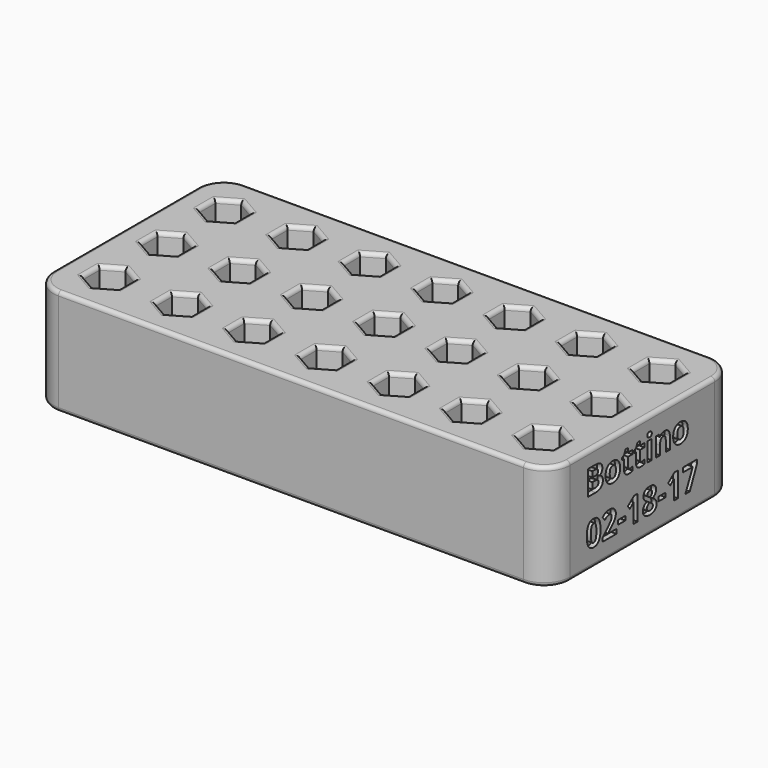
from build123d import *

# Parameters (mm, degrees)
F2_DEPTH     = 20.5
F3_DEPTH     = 12
F4_DEPTH     = 17
F5_R         = 0.5
F6_R         = 0.75
F7_TEXT_SIZE = 6.6788283418
F8_DEPTH     = 1


# Not quite as in the source:
# - Text() gives the source's letters only with a copy of the font that has no kerning and outlines rounded to 1/6400 em; it was checked with that copy


with BuildPart() as f2:
    # F1 (on Top) → F2 (new body)
    with BuildSketch(Plane.XY):
        with BuildLine():
            Line((45, 22.5), (-45, 22.5))
            ThreePointArc((-45, 22.5), (-48.5355339059, 21.0355339059), (-50, 17.5))
            Line((-50, 17.5), (-50, -17.5))
            ThreePointArc((-50, -17.5), (-48.5355339059, -21.0355339059), (-45, -22.5))
            Line((-45, -22.5), (45, -22.5))
            ThreePointArc((45, -22.5), (48.5355339059, -21.0355339059), (50, -17.5))
            Line((50, -17.5), (50, 17.5))
            ThreePointArc((50, 17.5), (48.5355339059, 21.0355339059), (45, 22.5))
        make_face()
    extrude(amount=-F2_DEPTH)

    # F0 (on Top) → F3 (cut)
    with BuildSketch(Plane.XY):
        Polygon((-42, -10.0451506561), (-45.425, -12.022575328), (-45.425, -15.977424672), (-42, -17.9548493439), (-38.575, -15.977424672), (-38.575, -12.022575328), align=None)
        Polygon((-28, -10.0451506561), (-31.425, -12.022575328), (-31.425, -15.977424672), (-28, -17.9548493439), (-24.575, -15.977424672), (-24.575, -12.022575328), align=None)
        Polygon((-14, -17.9548493439), (-10.575, -15.977424672), (-10.575, -12.022575328), (-14, -10.0451506561), (-17.425, -12.022575328), (-17.425, -15.977424672), align=None)
        Polygon((-3.425, -12.022575328), (-3.425, -15.977424672), (0, -17.9548493439), (3.425, -15.977424672), (3.425, -12.022575328), (0, -10.0451506561), align=None)
        Polygon((10.575, -12.022575328), (10.575, -15.977424672), (14, -17.9548493439), (17.425, -15.977424672), (17.425, -12.022575328), (14, -10.0451506561), align=None)
        Polygon((31.425, -12.022575328), (28, -10.0451506561), (24.575, -12.022575328), (24.575, -15.977424672), (28, -17.9548493439), (31.425, -15.977424672), align=None)
        Polygon((45.425, -12.022575328), (42, -10.0451506561), (38.575, -12.022575328), (38.575, -15.977424672), (42, -17.9548493439), (45.425, -15.977424672), align=None)
    extrude(amount=-F3_DEPTH, mode=Mode.SUBTRACT)

    # F0 (on Top) → F4 (cut)
    with BuildSketch(Plane.XY):
        Polygon((-38.575, 12.022575328), (-38.575, 15.977424672), (-42, 17.9548493439), (-45.425, 15.977424672), (-45.425, 12.022575328), (-42, 10.0451506561), align=None)
        Polygon((-28, 10.0451506561), (-24.575, 12.022575328), (-24.575, 15.977424672), (-28, 17.9548493439), (-31.425, 15.977424672), (-31.425, 12.022575328), align=None)
        Polygon((-10.575, 12.022575328), (-10.575, 15.977424672), (-14, 17.9548493439), (-17.425, 15.977424672), (-17.425, 12.022575328), (-14, 10.0451506561), align=None)
        Polygon((0, 17.9548493439), (-3.425, 15.977424672), (-3.425, 12.022575328), (0, 10.0451506561), (3.425, 12.022575328), (3.425, 15.977424672), align=None)
        Polygon((14, 17.9548493439), (10.575, 15.977424672), (10.575, 12.022575328), (14, 10.0451506561), (17.425, 12.022575328), (17.425, 15.977424672), align=None)
        Polygon((28, 17.9548493439), (24.575, 15.977424672), (24.575, 12.022575328), (28, 10.0451506561), (31.425, 12.022575328), (31.425, 15.977424672), align=None)
        Polygon((42, 17.9548493439), (38.575, 15.977424672), (38.575, 12.022575328), (42, 10.0451506561), (45.425, 12.022575328), (45.425, 15.977424672), align=None)
        Polygon((42, 3.9548493439), (38.575, 1.977424672), (38.575, -1.977424672), (42, -3.9548493439), (45.425, -1.977424672), (45.425, 1.977424672), align=None)
        Polygon((28, 3.9548493439), (24.575, 1.977424672), (24.575, -1.977424672), (28, -3.9548493439), (31.425, -1.977424672), (31.425, 1.977424672), align=None)
        Polygon((14, 3.9548493439), (10.575, 1.977424672), (10.575, -1.977424672), (14, -3.9548493439), (17.425, -1.977424672), (17.425, 1.977424672), align=None)
        Polygon((3.425, -1.977424672), (3.425, 1.977424672), (0, 3.9548493439), (-3.425, 1.977424672), (-3.425, -1.977424672), (0, -3.9548493439), align=None)
        Polygon((-10.575, -1.977424672), (-10.575, 1.977424672), (-14, 3.9548493439), (-17.425, 1.977424672), (-17.425, -1.977424672), (-14, -3.9548493439), align=None)
        Polygon((-24.575, 1.977424672), (-28, 3.9548493439), (-31.425, 1.977424672), (-31.425, -1.977424672), (-28, -3.9548493439), (-24.575, -1.977424672), align=None)
        Polygon((-38.575, -1.977424672), (-38.575, 1.977424672), (-42, 3.9548493439), (-45.425, 1.977424672), (-45.425, -1.977424672), (-42, -3.9548493439), align=None)
    extrude(amount=-F4_DEPTH, mode=Mode.SUBTRACT)

    # F5
    f5_edges = [f2.edges().sort_by_distance(p)[0] for p in [
        (-38.575, 14, -17),
        (-40.2875, 16.966137, -17),
        (-43.7125, 16.966137, -17),
        (-45.425, 14, -17),
        (-43.7125, 11.033863, -17),
        (-40.2875, 11.033863, -17),
        (-26.2875, 11.033863, -17),
        (-24.575, 14, -17),
        (-26.2875, 16.966137, -17),
        (-29.7125, 16.966137, -17),
        (-31.425, 14, -17),
        (-29.7125, 11.033863, -17),
        (-10.575, 14, -17),
        (-12.2875, 16.966137, -17),
        (-15.7125, 16.966137, -17),
        (-17.425, 14, -17),
        (-15.7125, 11.033863, -17),
        (-12.2875, 11.033863, -17),
        (-1.7125, 16.966137, -17),
        (-3.425, 14, -17),
        (-1.7125, 11.033863, -17),
        (1.7125, 11.033863, -17),
        (3.425, 14, -17),
        (1.7125, 16.966137, -17),
        (12.2875, 16.966137, -17),
        (10.575, 14, -17),
        (12.2875, 11.033863, -17),
        (15.7125, 11.033863, -17),
        (17.425, 14, -17),
        (15.7125, 16.966137, -17),
        (26.2875, 16.966137, -17),
        (24.575, 14, -17),
        (26.2875, 11.033863, -17),
        (29.7125, 11.033863, -17),
        (31.425, 14, -17),
        (29.7125, 16.966137, -17),
        (40.2875, 16.966137, -17),
        (38.575, 14, -17),
        (40.2875, 11.033863, -17),
        (43.7125, 11.033863, -17),
        (45.425, 14, -17),
        (43.7125, 16.966137, -17),
        (40.2875, 2.966137, -17),
        (38.575, 0, -17),
        (40.2875, -2.966137, -17),
        (43.7125, -2.966137, -17),
        (45.425, 0, -17),
        (43.7125, 2.966137, -17),
        (26.2875, 2.966137, -17),
        (24.575, 0, -17),
        (26.2875, -2.966137, -17),
        (29.7125, -2.966137, -17),
        (31.425, 0, -17),
        (29.7125, 2.966137, -17),
        (12.2875, 2.966137, -17),
        (10.575, 0, -17),
        (12.2875, -2.966137, -17),
        (15.7125, -2.966137, -17),
        (17.425, 0, -17),
        (15.7125, 2.966137, -17),
        (1.7125, -2.966137, -17),
        (3.425, 0, -17),
        (1.7125, 2.966137, -17),
        (-1.7125, 2.966137, -17),
        (-3.425, 0, -17),
        (-1.7125, -2.966137, -17),
        (-12.2875, -2.966137, -17),
        (-10.575, 0, -17),
        (-12.2875, 2.966137, -17),
        (-15.7125, 2.966137, -17),
        (-17.425, 0, -17),
        (-15.7125, -2.966137, -17),
        (-24.575, 0, -17),
        (-26.2875, 2.966137, -17),
        (-29.7125, 2.966137, -17),
        (-31.425, 0, -17),
        (-29.7125, -2.966137, -17),
        (-26.2875, -2.966137, -17),
        (-38.575, 0, -17),
        (-40.2875, 2.966137, -17),
        (-43.7125, 2.966137, -17),
        (-45.425, 0, -17),
        (-43.7125, -2.966137, -17),
        (-40.2875, -2.966137, -17),
        (-40.2875, -11.033863, -12),
        (-43.7125, -11.033863, -12),
        (-45.425, -14, -12),
        (-43.7125, -16.966137, -12),
        (-40.2875, -16.966137, -12),
        (-38.575, -14, -12),
        (-26.2875, -11.033863, -12),
        (-29.7125, -11.033863, -12),
        (-31.425, -14, -12),
        (-29.7125, -16.966137, -12),
        (-26.2875, -16.966137, -12),
        (-24.575, -14, -12),
        (-12.2875, -16.966137, -12),
        (-10.575, -14, -12),
        (-12.2875, -11.033863, -12),
        (-15.7125, -11.033863, -12),
        (-17.425, -14, -12),
        (-15.7125, -16.966137, -12),
        (-3.425, -14, -12),
        (-1.7125, -16.966137, -12),
        (1.7125, -16.966137, -12),
        (3.425, -14, -12),
        (1.7125, -11.033863, -12),
        (-1.7125, -11.033863, -12),
        (10.575, -14, -12),
        (12.2875, -16.966137, -12),
        (15.7125, -16.966137, -12),
        (17.425, -14, -12),
        (15.7125, -11.033863, -12),
        (12.2875, -11.033863, -12),
        (29.7125, -16.966137, -12),
        (31.425, -14, -12),
        (29.7125, -11.033863, -12),
        (26.2875, -11.033863, -12),
        (24.575, -14, -12),
        (26.2875, -16.966137, -12),
        (43.7125, -16.966137, -12),
        (45.425, -14, -12),
        (43.7125, -11.033863, -12),
        (40.2875, -11.033863, -12),
        (38.575, -14, -12),
        (40.2875, -16.966137, -12),
    ]]
    fillet(f5_edges, radius=F5_R)

    # F6
    f6_edges = [f2.edges().sort_by_distance(p)[0] for p in [
        (-43.7125, 16.966137, 0),
        (-40.2875, 16.966137, 0),
        (-38.575, 14, 0),
        (-40.2875, 11.033863, 0),
        (-43.7125, 11.033863, 0),
        (-45.425, 14, 0),
        (-43.7125, 2.966137, 0),
        (-38.575, 0, 0),
        (-43.7125, -2.966137, 0),
        (-45.425, 0, 0),
        (-40.2875, 2.966137, 0),
        (-40.2875, -2.966137, 0),
        (-43.7125, -16.966137, 0),
        (-40.2875, -11.033863, 0),
        (-40.2875, -16.966137, 0),
        (-45.425, -14, 0),
        (-38.575, -14, 0),
        (-43.7125, -11.033863, 0),
        (-26.2875, -11.033863, 0),
        (-31.425, -14, 0),
        (-29.7125, -16.966137, 0),
        (-29.7125, -11.033863, 0),
        (-26.2875, -16.966137, 0),
        (-24.575, -14, 0),
        (-24.575, 0, 0),
        (-31.425, 0, 0),
        (-31.425, 14, 0),
        (-26.2875, 16.966137, 0),
        (-26.2875, 2.966137, 0),
        (-26.2875, 11.033863, 0),
        (-29.7125, 16.966137, 0),
        (-29.7125, 11.033863, 0),
        (-29.7125, 2.966137, 0),
        (-26.2875, -2.966137, 0),
        (-24.575, 14, 0),
        (-29.7125, -2.966137, 0),
        (-12.2875, -11.033863, 0),
        (-12.2875, -16.966137, 0),
        (-17.425, -14, 0),
        (-12.2875, 2.966137, 0),
        (-12.2875, 11.033863, 0),
        (-12.2875, -2.966137, 0),
        (-15.7125, 16.966137, 0),
        (-12.2875, 16.966137, 0),
        (-17.425, 0, 0),
        (-17.425, 14, 0),
        (-10.575, 14, 0),
        (-10.575, 0, 0),
        (-15.7125, -16.966137, 0),
        (-15.7125, -11.033863, 0),
        (-10.575, -14, 0),
        (-15.7125, -2.966137, 0),
        (-15.7125, 2.966137, 0),
        (-15.7125, 11.033863, 0),
        (-1.7125, 16.966137, 0),
        (1.7125, 16.966137, 0),
        (-3.425, 14, 0),
        (3.425, -14, 0),
        (1.7125, -11.033863, 0),
        (-1.7125, -11.033863, 0),
        (-3.425, -14, 0),
        (12.2875, -11.033863, 0),
        (12.2875, 16.966137, 0),
        (15.7125, 11.033863, 0),
        (-3.425, 0, 0),
        (12.2875, -16.966137, 0),
        (1.7125, -2.966137, 0),
        (3.425, 14, 0),
        (15.7125, 2.966137, 0),
        (17.425, 0, 0),
        (12.2875, 11.033863, 0),
        (10.575, 14, 0),
        (12.2875, 2.966137, 0),
        (1.7125, 11.033863, 0),
        (-1.7125, -16.966137, 0),
        (17.425, 14, 0),
        (-1.7125, 11.033863, 0),
        (15.7125, 16.966137, 0),
        (-1.7125, 2.966137, 0),
        (10.575, -14, 0),
        (3.425, 0, 0),
        (-1.7125, -2.966137, 0),
        (15.7125, -16.966137, 0),
        (15.7125, -11.033863, 0),
        (1.7125, -16.966137, 0),
        (12.2875, -2.966137, 0),
        (17.425, -14, 0),
        (10.575, 0, 0),
        (15.7125, -2.966137, 0),
        (1.7125, 2.966137, 0),
        (-45, -22.5, -10.25),
        (45, -22.5, -10.25),
        (0, -22.5, 0),
        (0, -22.5, -20.5),
        (43.7125, -16.966137, 0),
        (38.575, 14, 0),
        (31.425, 14, 0),
        (40.2875, 2.966137, 0),
        (38.575, -14, 0),
        (31.425, 0, 0),
        (24.575, 0, 0),
        (29.7125, -11.033863, 0),
        (29.7125, 16.966137, 0),
        (26.2875, -16.966137, 0),
        (26.2875, 2.966137, 0),
        (40.2875, 16.966137, 0),
        (29.7125, -16.966137, 0),
        (26.2875, 16.966137, 0),
        (43.7125, -2.966137, 0),
        (29.7125, -2.966137, 0),
        (24.575, 14, 0),
        (40.2875, -11.033863, 0),
        (38.575, 0, 0),
        (40.2875, -16.966137, 0),
        (40.2875, -2.966137, 0),
        (26.2875, -2.966137, 0),
        (45.425, 0, 0),
        (26.2875, 11.033863, 0),
        (45.425, 14, 0),
        (45.425, -14, 0),
        (31.425, -14, 0),
        (26.2875, -11.033863, 0),
        (43.7125, 11.033863, 0),
        (24.575, -14, 0),
        (43.7125, 2.966137, 0),
        (43.7125, 16.966137, 0),
        (29.7125, 11.033863, 0),
        (29.7125, 2.966137, 0),
        (40.2875, 11.033863, 0),
        (43.7125, -11.033863, 0),
    ]]
    fillet(f6_edges, radius=F6_R)

    # F7 (on face) → F8 (cut)
    with BuildSketch(Plane.YZ.offset(50)):
        with Locations((-13.6957723683, -7.8845415196)):
            Text('Bottino', F7_TEXT_SIZE, font='Open Sans', font_style=FontStyle.BOLD, text_align=(TextAlign.LEFT, TextAlign.BOTTOM))
        with Locations((-13.6957723683, -16.9677480644)):
            Text('02-18-17', F7_TEXT_SIZE, font='Open Sans', font_style=FontStyle.BOLD, text_align=(TextAlign.LEFT, TextAlign.BOTTOM))
    extrude(amount=-F8_DEPTH, mode=Mode.SUBTRACT)


solid = f2.part
